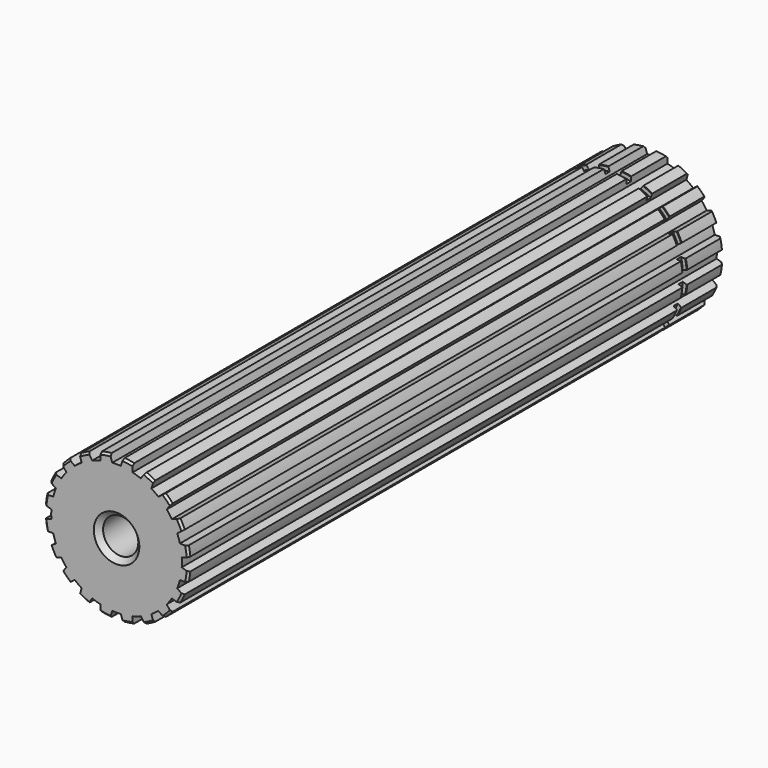
from build123d import *

# Parameters (mm, degrees)
F1_DEPTH        = 161.5
F3_D            = 16
F3_DEPTH        = 31
F3_CSINK_D      = 17
F3_CSINK_ANGLE  = 90
F3_TIP          = 4.8068849522
F2_R            = 11
F4_DEPTH        = 25
F6_R            = 17.5
F6_R_2          = 16.45
F7_DEPTH        = 1.3
F8_SIZE         = 0.5
F9_R            = 0.2
F10_SIZE        = 0.1
F12_D           = 8.5
F12_DEPTH       = 40
F12_CSINK_D     = 11
F12_CSINK_ANGLE = 90
F12_TIP         = 2.5536576309


# Not quite as in the source:
# - ends of sketch curves that miss each other by under 0.0002 mm in the source are joined


with BuildPart() as f1:
    # F0 (on Front) → F1 (new body)
    with BuildSketch(Plane.XZ):
        with BuildLine():
            Line((-6.887924, -16.081209), (-5.851508, -14.654705))
            ThreePointArc((-5.851508, -14.654705), (-4.8762111235, -15.0074339959), (-3.87985001, -15.2953350392))
            Line((-3.87985001, -15.2953350392), (-3.87985, -17.058592))
            ThreePointArc((-3.87985, -17.058592), (-2.7367040616, -17.2788666857), (-1.5814390173, -17.4226241909))
            Line((-1.5814390173, -17.4226241909), (-1.036562, -15.745668))
            ThreePointArc((-1.036562, -15.745668), (0, -15.77975), (1.0365619761, -15.7456676369))
            Line((1.0365619761, -15.7456676369), (1.581438, -17.422625))
            ThreePointArc((1.581438, -17.422625), (2.7367035697, -17.2788667636), (3.8798499114, -17.0585916103))
            Line((3.8798499114, -17.0585916103), (3.87985, -15.295335))
            ThreePointArc((3.87985, -15.295335), (4.8762106819, -15.0074341394), (5.8515073121, -14.6547047817))
            Line((5.8515073121, -14.6547047817), (6.887924, -16.081209))
            ThreePointArc((6.887924, -16.081209), (7.942223228, -15.5874909225), (8.9613511318, -15.024745221))
            Line((8.9613511318, -15.024745221), (8.416475, -13.347789))
            ThreePointArc((8.416475, -13.347789), (9.2751042792, -12.7660859574), (10.0936671288, -12.1292371547))
            Line((10.0936671288, -12.1292371547), (11.520172, -13.165654))
            ThreePointArc((11.520172, -13.165654), (12.3703028068, -12.3703028068), (13.1656530266, -11.5201720233))
            Line((13.1656530266, -11.5201720233), (12.129237, -10.093668))
            ThreePointArc((12.129237, -10.093668), (12.7660859574, -9.2751042792), (13.3477883791, -8.416475239))
            Line((13.3477883791, -8.416475239), (15.024745, -8.961352))
            ThreePointArc((15.024745, -8.961352), (15.5874909225, -7.942223228), (16.0812090823, -6.8879240352))
            Line((16.0812090823, -6.8879240352), (14.654704, -5.851508))
            ThreePointArc((14.654704, -5.851508), (15.0074339959, -4.8762111235), (15.2953350392, -3.87985001))
            Line((15.2953350392, -3.87985001), (17.058591, -3.87985))
            ThreePointArc((17.058591, -3.87985), (17.2788667462, -2.7367036793), (17.4226242809, -1.5814380255))
            Line((17.4226242809, -1.5814380255), (15.745667, -1.036562))
            ThreePointArc((15.745667, -1.036562), (15.77975, 0), (15.7456676326, 1.0365620416))
            Line((15.7456676326, 1.0365620416), (17.422624, 1.581438))
            ThreePointArc((17.422624, 1.581438), (17.2788667462, 2.7367036793), (17.0585915611, 3.8798501276))
            Line((17.0585915611, 3.8798501276), (15.295335, 3.87985))
            ThreePointArc((15.295335, 3.87985), (15.0074339959, 4.8762111235), (14.6547044373, 5.8515081746))
            Line((14.6547044373, 5.8515081746), (16.081209, 6.887924))
            ThreePointArc((16.081209, 6.887924), (15.5874909225, 7.942223228), (15.024745221, 8.9613511318))
            Line((15.024745221, 8.9613511318), (13.347788, 8.416475))
            ThreePointArc((13.347788, 8.416475), (12.7660857315, 9.2751045902), (12.1292366631, 10.0936677196))
            Line((12.1292366631, 10.0936677196), (13.165653, 11.520172))
            ThreePointArc((13.165653, 11.520172), (12.3703028068, 12.3703028068), (11.5201720233, 13.1656530266))
            Line((11.5201720233, 13.1656530266), (10.093667, 12.129237))
            ThreePointArc((10.093667, 12.129237), (9.2751040635, 12.7660861142), (8.4164747879, 13.3477886636))
            Line((8.4164747879, 13.3477886636), (8.961351, 15.024745))
            ThreePointArc((8.961351, 15.024745), (7.942223228, 15.5874909225), (6.8879240352, 16.0812090823))
            Line((6.8879240352, 16.0812090823), (5.851507, 14.654704))
            ThreePointArc((5.851507, 14.654704), (4.8762105056, 15.0074341967), (3.87985001, 15.2953350392))
            Line((3.87985001, 15.2953350392), (3.87985, 17.058591))
            ThreePointArc((3.87985, 17.058591), (2.7367035697, 17.2788667636), (1.5814380255, 17.4226242809))
            Line((1.5814380255, 17.4226242809), (1.036561, 15.745667))
            ThreePointArc((1.036561, 15.745667), (0, 15.77975), (-1.0365619761, 15.7456676369))
            Line((-1.0365619761, 15.7456676369), (-1.581438, 17.422624))
            ThreePointArc((-1.581438, 17.422624), (-2.7367040616, 17.2788666857), (-3.8798499114, 17.0585916103))
            Line((-3.8798499114, 17.0585916103), (-3.87985, 15.295335))
            ThreePointArc((-3.87985, 15.295335), (-4.8762109472, 15.0074340532), (-5.8515078302, 14.6547045748))
            Line((-5.8515078302, 14.6547045748), (-6.887924, 16.081209))
            ThreePointArc((-6.887924, 16.081209), (-7.9422236106, 15.5874907276), (-8.9613518694, 15.024744781))
            Line((-8.9613518694, 15.024744781), (-8.416475, 13.347788))
            ThreePointArc((-8.416475, 13.347788), (-9.2751043744, 12.7660858883), (-10.0936677196, 12.1292366631))
            Line((-10.0936677196, 12.1292366631), (-11.520172, 13.165653))
            ThreePointArc((-11.520172, 13.165653), (-12.3703028068, 12.3703028068), (-13.1656530266, 11.5201720233))
            Line((-13.1656530266, 11.5201720233), (-12.129237, 10.093667))
            ThreePointArc((-12.129237, 10.093667), (-12.7660858883, 9.2751043744), (-13.3477886636, 8.4164747879))
            Line((-13.3477886636, 8.4164747879), (-15.024745, 8.961351))
            ThreePointArc((-15.024745, 8.961351), (-15.5874910388, 7.9422229997), (-16.0812090823, 6.8879240352))
            Line((-16.0812090823, 6.8879240352), (-14.654705, 5.851507))
            ThreePointArc((-14.654705, 5.851507), (-15.0074340532, 4.8762109472), (-15.2953350392, 3.87985001))
            Line((-15.2953350392, 3.87985001), (-17.058592, 3.87985))
            ThreePointArc((-17.058592, 3.87985), (-17.2788667707, 2.7367035251), (-17.4226242891, 1.5814379355))
            Line((-17.4226242891, 1.5814379355), (-15.745668, 1.036561))
            ThreePointArc((-15.745668, 1.036561), (-15.77975, 0), (-15.7456676369, -1.0365619761))
            Line((-15.7456676369, -1.0365619761), (-17.422625, -1.581438))
            ThreePointArc((-17.422625, -1.581438), (-17.2788667707, -2.7367035251), (-17.0585916103, -3.8798499114))
            Line((-17.0585916103, -3.8798499114), (-15.295335, -3.87985))
            ThreePointArc((-15.295335, -3.87985), (-15.0074340532, -4.8762109472), (-14.6547045748, -5.8515078302))
            Line((-14.6547045748, -5.8515078302), (-16.081209, -6.887924))
            ThreePointArc((-16.081209, -6.887924), (-15.5874910388, -7.9422229997), (-15.0247454834, -8.9613506919))
            Line((-15.0247454834, -8.9613506919), (-13.347789, -8.416475))
            ThreePointArc((-13.347789, -8.416475), (-12.7660861142, -9.2751040635), (-12.1292371547, -10.0936671288))
            Line((-12.1292371547, -10.0936671288), (-13.165654, -11.520172))
            ThreePointArc((-13.165654, -11.520172), (-12.3703028068, -12.3703028068), (-11.5201720233, -13.1656530266))
            Line((-11.5201720233, -13.1656530266), (-10.093668, -12.129237))
            ThreePointArc((-10.093668, -12.129237), (-9.2751045902, -12.7660857315), (-8.416475239, -13.3477883791))
            Line((-8.416475239, -13.3477883791), (-8.961352, -15.024745))
            ThreePointArc((-8.961352, -15.024745), (-7.9422236106, -15.5874907276), (-6.887924, -16.081209))
        make_face()
    extrude(amount=-F1_DEPTH)

    # F3
    with Locations(Plane(origin=(0, 161.5, 0), x_dir=(-1, 0, 0), z_dir=(0, 1, 0))):
        with Locations((0, 0)):
            CounterSinkHole(F3_D / 2, F3_CSINK_D / 2, depth=F3_DEPTH, counter_sink_angle=F3_CSINK_ANGLE)
            with Locations((0, 0, -(F3_DEPTH + F3_TIP / 2))):  # 118° drill point
                Cone(0, F3_D / 2, F3_TIP, mode=Mode.SUBTRACT)

    # F2 (on face) → F4 (cut)
    with BuildSketch(Plane(origin=(0, 161.5, 0), x_dir=(-1, 0, 0), z_dir=(0, 1, 0))):
        Circle(F2_R)
    extrude(amount=-F4_DEPTH, mode=Mode.SUBTRACT)

    # F6 (on offset) → F7 (cut)
    with BuildSketch(Plane(origin=(0, 150.4574, 0), x_dir=(-1, 0, 0), z_dir=(0, 1, 0))):
        Circle(F6_R)
        Circle(F6_R_2, mode=Mode.SUBTRACT)
    extrude(amount=-F7_DEPTH, mode=Mode.SUBTRACT)

    # F8
    f8_edges = [f1.edges().sort_by_distance(p)[0] for p in [
        (11, 161.5, 0),
        (7.942223, 161.5, 15.587491),
        (2.736704, 161.5, 17.278867),
        (-2.736704, 161.5, 17.278867),
        (12.370303, 161.5, 12.370303),
        (15.587491, 161.5, 7.942223),
        (17.278867, 161.5, 2.736704),
        (-7.942224, 161.5, 15.587491),
        (-12.370303, 161.5, 12.370303),
        (-15.587491, 161.5, 7.942223),
        (-17.278867, 161.5, 2.736704),
        (-17.278867, 161.5, -2.736704),
        (-15.587491, 161.5, -7.942223),
        (-12.370303, 161.5, -12.370303),
        (-7.942224, 161.5, -15.587491),
        (-2.736704, 161.5, -17.278867),
        (2.736704, 161.5, -17.278867),
        (7.942223, 161.5, -15.587491),
        (12.370303, 161.5, -12.370303),
        (15.587491, 161.5, -7.942224),
        (17.278867, 161.5, -2.736704),
        (-12.370303, 0, 12.370303),
        (-7.942224, 0, 15.587491),
        (-2.736704, 0, 17.278867),
        (-15.587491, 0, 7.942223),
        (2.736704, 0, 17.278867),
        (7.942223, 0, 15.587491),
        (12.370303, 0, 12.370303),
        (15.587491, 0, 7.942223),
        (17.278867, 0, 2.736704),
        (17.278867, 0, -2.736704),
        (15.587491, 0, -7.942224),
        (12.370303, 0, -12.370303),
        (7.942223, 0, -15.587491),
        (2.736704, 0, -17.278867),
        (-2.736704, 0, -17.278867),
        (-7.942224, 0, -15.587491),
        (-12.370303, 0, -12.370303),
        (-15.587491, 0, -7.942223),
        (-17.278867, 0, -2.736704),
        (-17.278867, 0, 2.736704),
        (8, 136.5, 0),
    ]]
    chamfer(f8_edges, length=F8_SIZE)

    # F9
    f9_edges = [f1.edges().sort_by_distance(p)[0] for p in [
        (11, 136.5, 0),
    ]]
    fillet(f9_edges, radius=F9_R)

    # F10
    f10_edges = [f1.edges().sort_by_distance(p)[0] for p in [
        (12.370303, 149.1574, 12.370303),
        (7.942223, 149.1574, 15.587491),
        (15.587491, 149.1574, 7.942223),
        (2.736704, 149.1574, 17.278867),
        (17.278867, 149.1574, 2.736704),
        (-2.736704, 149.1574, 17.278867),
        (17.278867, 149.1574, -2.736704),
        (-7.942224, 149.1574, 15.587491),
        (15.587491, 149.1574, -7.942224),
        (-12.370303, 149.1574, 12.370303),
        (12.370303, 149.1574, -12.370303),
        (-15.587491, 149.1574, 7.942223),
        (7.942223, 149.1574, -15.587491),
        (-17.278867, 149.1574, 2.736704),
        (2.736704, 149.1574, -17.278867),
        (-17.278867, 149.1574, -2.736704),
        (-2.736704, 149.1574, -17.278867),
        (-15.587491, 149.1574, -7.942223),
        (-7.942224, 149.1574, -15.587491),
        (-12.370303, 149.1574, -12.370303),
        (12.370303, 150.4574, 12.370303),
        (7.942223, 150.4574, 15.587491),
        (15.587491, 150.4574, 7.942223),
        (2.736704, 150.4574, 17.278867),
        (17.278867, 150.4574, 2.736704),
        (-2.736704, 150.4574, 17.278867),
        (17.278867, 150.4574, -2.736704),
        (-7.942224, 150.4574, 15.587491),
        (15.587491, 150.4574, -7.942224),
        (-12.370303, 150.4574, 12.370303),
        (12.370303, 150.4574, -12.370303),
        (-15.587491, 150.4574, 7.942223),
        (7.942223, 150.4574, -15.587491),
        (-17.278867, 150.4574, 2.736704),
        (2.736704, 150.4574, -17.278867),
        (-17.278867, 150.4574, -2.736704),
        (-2.736704, 150.4574, -17.278867),
        (-15.587491, 150.4574, -7.942223),
        (-7.942224, 150.4574, -15.587491),
        (-12.370303, 150.4574, -12.370303),
    ]]
    chamfer(f10_edges, length=F10_SIZE)

    # F12
    with Locations(Plane.XZ):
        with Locations((0, 0)):
            CounterSinkHole(F12_D / 2, F12_CSINK_D / 2, depth=F12_DEPTH, counter_sink_angle=F12_CSINK_ANGLE)
            with Locations((0, 0, -(F12_DEPTH + F12_TIP / 2))):  # 118° drill point
                Cone(0, F12_D / 2, F12_TIP, mode=Mode.SUBTRACT)


solid = f1.part
